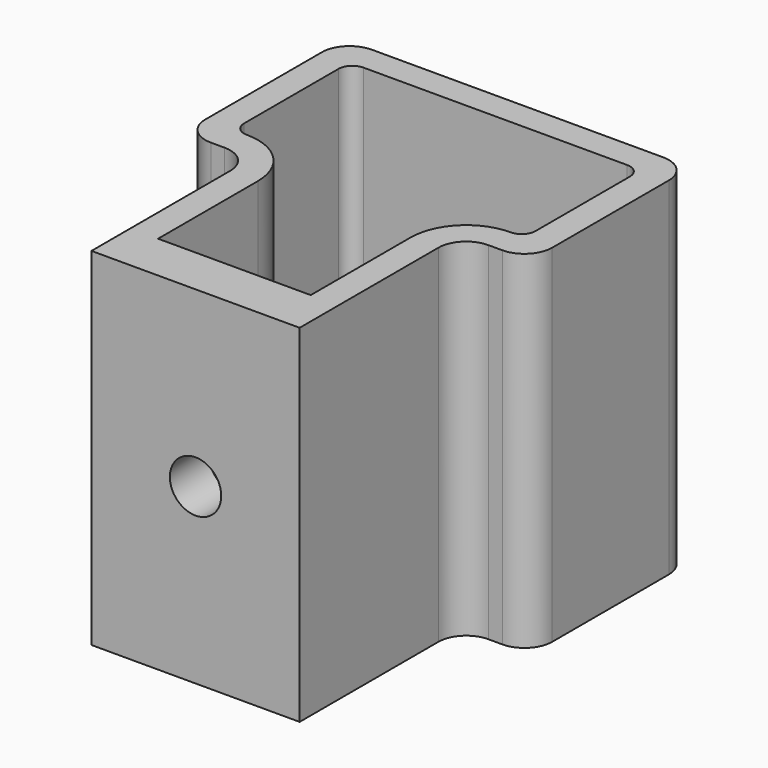
from build123d import *

# Parameters (mm, degrees)
F1_DEPTH    = 25
F2_R        = 1.85
F3_DEPTH    = 16.3
F4_T1_DEPTH = 25
F7_R        = 4
F5_DEPTH    = 8.1194955856
F6_DEPTH    = 1.5


# Not quite as in the source:
# - a fillet or chamfer that OpenCascade refuses, or shapes differently, is made with other operations: its cross-section is extruded or revolved along the edge and cut away or added


with BuildPart() as f1:
    # F0 (on Top) → F1 (new body)
    with BuildSketch(Plane.XY):
        with BuildLine():
            Line((-7.5, -2), (-7.5, -14.5))
            Line((-7.5, -14.5), (7.5, -14.5))
            Line((7.5, -14.5), (7.5, -2))
            ThreePointArc((7.5, -2), (8.0857864376, -0.5857864376), (9.5, 0))
            Line((9.5, 0), (10.5, 0))
            ThreePointArc((10.5, 0), (11.9142135624, 0.5857864376), (12.5, 2))
            Line((12.5, 2), (12.5, 12.5))
            ThreePointArc((12.5, 12.5), (11.9142135624, 13.9142135624), (10.5, 14.5))
            Line((10.5, 14.5), (-10.5, 14.5))
            ThreePointArc((-10.5, 14.5), (-11.9142135624, 13.9142135624), (-12.5, 12.5))
            Line((-12.5, 12.5), (-12.5, 2))
            ThreePointArc((-12.5, 2), (-11.9142135624, 0.5857864376), (-10.5, 0))
            Line((-10.5, 0), (-9.5, 0))
            ThreePointArc((-9.5, 0), (-8.0857864376, -0.5857864376), (-7.5, -2))
        make_face()
        with BuildLine():
            Line((-10.5, 1.8729833462), (-10.5, 12.5))
            Line((-10.5, 12.5), (10.5, 12.5))
            Line((10.5, 12.5), (10.5, 1.8729833462))
            ThreePointArc((10.5, 1.8729833462), (7.0505102572, 1.1622776602), (5.5, -2))
            Line((5.5, -2), (5.5, -12.5))
            Line((5.5, -12.5), (-5.5, -12.5))
            Line((-5.5, -12.5), (-5.5, -2))
            ThreePointArc((-5.5, -2), (-7.0505102572, 1.1622776602), (-10.5, 1.8729833462))
        make_face(mode=Mode.SUBTRACT)
    extrude(amount=F1_DEPTH)

    # F2 (on face) → F3 (cut)
    with BuildSketch(Plane.XZ.offset(14.5)):
        with Locations((0, 12.5)):
            Circle(F2_R)
    extrude(amount=-F3_DEPTH, mode=Mode.SUBTRACT)

    # F4: fillet of radius 1 on 4 edges, made by hand

    # F4_s2 → F4_t1 (join)
    with BuildSketch(Plane.XY):
        with BuildLine():
            ThreePointArc((-10.5, 11.5), (-10.2071067812, 12.2071067812), (-9.5, 12.5))
            Line((-9.5, 12.5), (-10.5, 12.5))
            Line((-10.5, 12.5), (-10.5, 11.5))
        make_face()
        with BuildLine():
            ThreePointArc((9.5, 12.5), (10.2071067812, 12.2071067812), (10.5, 11.5))
            Line((10.5, 11.5), (10.5, 12.5))
            Line((10.5, 12.5), (9.5, 12.5))
        make_face()
        with BuildLine():
            ThreePointArc((9.5, 2), (10.2071067812, 2.2928932188), (10.5, 3))
            Line((10.5, 3), (10.5, 1.8729833462))
            ThreePointArc((10.5, 1.8729833462), (10.0040171699, 1.9681187851), (9.5, 2))
        make_face()
        with BuildLine():
            ThreePointArc((-9.5, 2), (-10.2071067812, 2.2928932188), (-10.5, 3))
            Line((-10.5, 3), (-10.5, 1.8729833462))
            ThreePointArc((-10.5, 1.8729833462), (-10.0040171699, 1.9681187851), (-9.5, 2))
        make_face()
    extrude(amount=F4_T1_DEPTH)

    # F7 (on face) → F5 (cut)
    with BuildSketch(Plane(origin=(0, 14.5, 0), x_dir=(-1, 0, 0), z_dir=(0, 1, 0))):
        with Locations((0, 12.5)):
            Circle(F7_R)
    extrude(amount=-F5_DEPTH, mode=Mode.SUBTRACT)

    # F6 (add): a face of the model
    f6_faces = [f1.faces().sort_by_distance(p)[0] for p in [
        (5.2268699943, -12.5, 12.5),
    ]]
    extrude(f6_faces, amount=F6_DEPTH)


solid = f1.part
